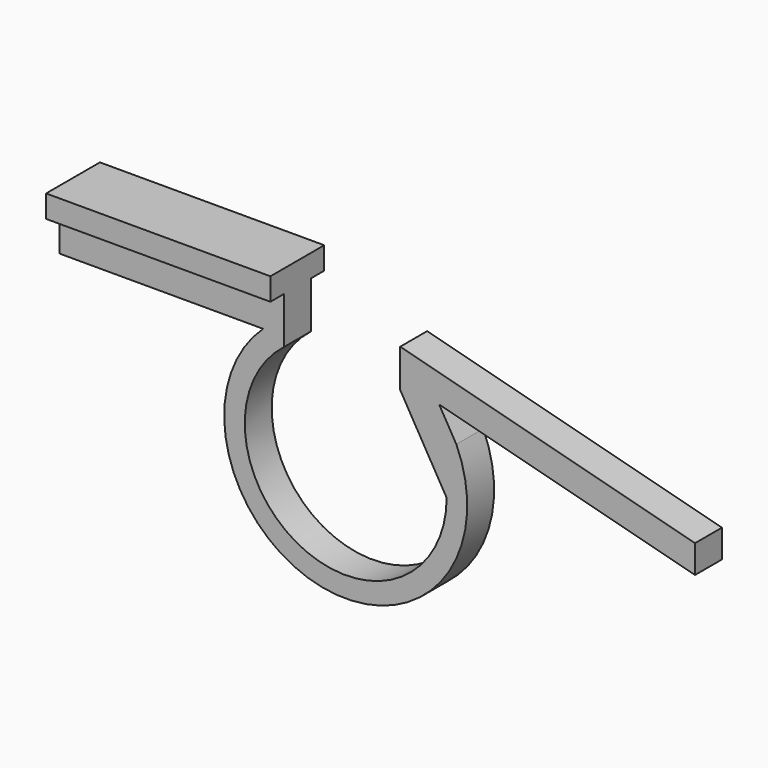
from build123d import *

# Parameters (mm, degrees)
F1_DEPTH = 1.143
F2_DEPTH = 1.143
F4_DEPTH = 15.24


# Not quite as in the source:
# - a feature names something its author has since deleted; it is built from what else it names


with BuildPart() as f1:
    # F0 (on Front) → F1 (new body, symmetric)
    with BuildSketch(Plane.XZ):
        with BuildLine():
            Line((0, 2.597206724), (0, 0))
            Line((0, 0), (3.1534308471, -5.4197111054))
            ThreePointArc((3.1534308471, -5.4197111054), (-6.7222786548, -11.5780869759), (-7.9068180192, 0))
            Line((-7.9068180192, 0), (-7.9068180192, 0.635))
            Line((-7.9068180192, 0.635), (-9.3157631818, 0.635))
            ThreePointArc((-9.3157631818, 0.635), (-5.3307842554, -13.5129459), (3.8098860109, -2.0024038921))
            Line((3.8098860109, -2.0024038921), (2.6447976734, 0))
            Line((2.6447976734, 0), (20.0257543474, -4.549011518))
            Line((20.0257543474, -4.549011518), (20.0257543474, -2.644011518))
            Line((20.0257543474, -2.644011518), (0, 2.597206724))
        make_face()
    extrude(amount=F1_DEPTH, both=True)

    # F0 (on Front) → F2 (join, symmetric)
    with BuildSketch(Plane.XZ):
        Polygon((-9.3157631818, 0.635), (-7.9068180192, 0.635), (-7.9068180192, 3.175), (-23.1468180192, 3.175), (-23.1468180192, 0.635), align=None)
    extrude(amount=F2_DEPTH, both=True)

    # F3 (on face) → F4 (join, through all)
    with BuildSketch(Plane(origin=(-23.1468180192, 0, 0), x_dir=(0, -1, 0), z_dir=(-1, 0, 0))):
        Polygon((-2.286, 4.699), (-2.286, 3.175), (0, 3.175), (2.286, 3.175), (2.286, 4.699), (0, 4.699), align=None)
    extrude(amount=-F4_DEPTH)


solid = f1.part
